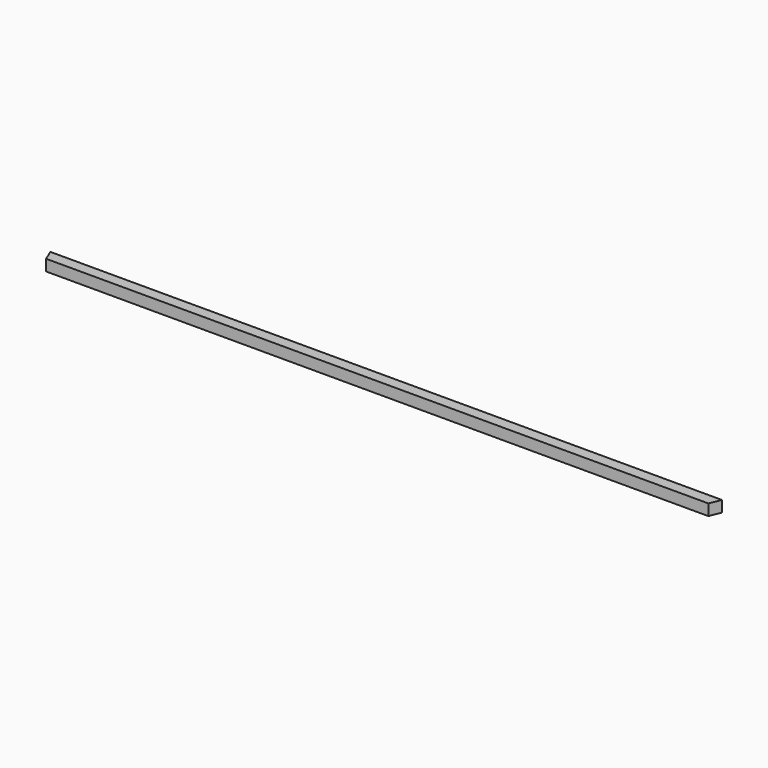
from build123d import *

# Parameters (mm, degrees)
F0_W       = 25.4
F0_H       = 25.4
F1_DEPTH   = 762
F2_SIZE2   = 10.521014
F2_SIZE    = 25.39999
F2_2_SIZE2 = 10.521014
F2_2_SIZE  = 25.39999


# Not quite as in the source:
# - a fillet or chamfer is up to 0.001 mm smaller than in the source, because OpenCascade refuses the exact size


with BuildPart() as f1:
    # F0 (on Right) → F1 (new body, symmetric)
    with BuildSketch(Plane.YZ):
        Rectangle(F0_W, F0_H)
    extrude(amount=F1_DEPTH, both=True)

    # F2 (size 25.4 and 10.5210244843 in the source; OpenCascade refuses exactly that, so slightly less here)
    f2_edges = [f1.edges().sort_by_distance(p)[0] for p in [
        (762, -12.7, 0),
    ]]
    f2_side = f1.faces().sort_by_distance((762, 0, 0))[0]
    chamfer(f2_edges, length=F2_SIZE, length2=F2_SIZE2, reference=f2_side)

    # F2#2 (size 25.4 and 10.5210244843 in the source; OpenCascade refuses exactly that, so slightly less here)
    f2_2_edges = [f1.edges().sort_by_distance(p)[0] for p in [
        (-762, -12.7, 0),
    ]]
    f2_2_side = f1.faces().sort_by_distance((-762, 0, 0))[0]
    chamfer(f2_2_edges, length=F2_2_SIZE, length2=F2_2_SIZE2, reference=f2_2_side)


solid = f1.part
